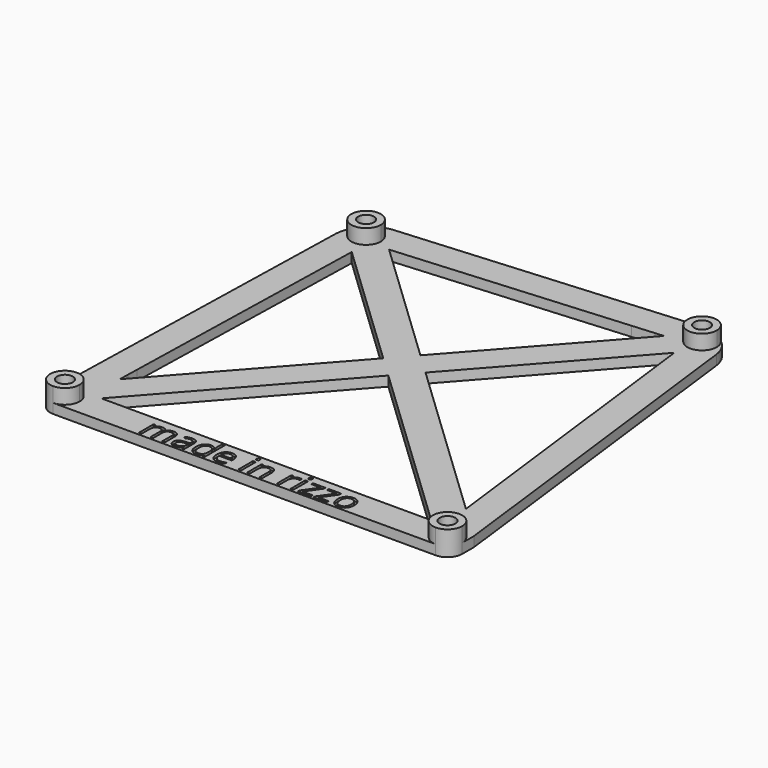
from build123d import *

# Parameters (mm, degrees)
F0_R         = 1.6
F1_DEPTH     = 2
F2_DEPTH     = 5
F3_TEXT_SIZE = 6.9444444444
F4_DEPTH     = 0.5
F5_T1_DEPTH  = 17
F6_R         = 6


# Not quite as in the source:
# - a fillet or chamfer that OpenCascade refuses, or shapes differently, is made with other operations: its cross-section is extruded or revolved along the edge and cut away or added
# - Text() gives the source's letters only with a copy of the font that has no kerning and outlines rounded to 1/6400 em; it was checked with that copy


with BuildPart() as f1:
    # F0 (on Top) → F1 (new body)
    with BuildSketch(Plane.XY):
        with BuildLine():
            ThreePointArc((-28.2406208698, -22.2661183476), (-29.1193005262, -24.3874386912), (-31.2406208698, -25.2661183476))
            Line((-31.2406208698, -25.2661183476), (46.7593791156, -25.2661183476))
            ThreePointArc((46.7593791156, -25.2661183476), (44.6380587918, -20.1447979989), (49.7593791302, -22.2661183476))
            Line((49.7593791302, -22.2661183476), (49.7593791302, -19.2661183476))
            Line((49.7593791302, -19.2661183476), (40.4943682456, 55.9885720374))
            Line((40.4943682456, 55.9885720374), (38.2495285372, 57.9787213655))
            Line((38.2495285372, 57.9787213655), (36.0046887452, 59.9688707678))
            Line((36.0046887452, 59.9688707678), (-28.3482573611, 54.975156742))
            Line((-28.3482573611, 54.975156742), (-30.4150766022, 52.8007010126))
            Line((-30.4150766022, 52.8007010126), (-32.4818959594, 50.626245161))
            Line((-32.4818959594, 50.626245161), (-34.2406208698, -19.2661183476))
            Line((-34.2406208698, -19.2661183476), (-34.2406208698, -22.2661183476))
            ThreePointArc((-34.2406208698, -22.2661183476), (-31.2406208698, -19.2661183476), (-28.2406208698, -22.2661183476))
        make_face()
        Polygon((0.1904056561, 19.5712364447), (-28.0633893681, -12.2983524785), (-28.0115448824, -10.2380338825), (-27.9546075256, -7.9753227447), (-26.6201953034, 45.0547011937), align=None, mode=Mode.SUBTRACT)
        Polygon((41.0503449115, -19.2661183476), (-26.2222311392, -19.2661183476), (4.5419359349, 15.4351087752), align=None, mode=Mode.SUBTRACT)
        with BuildLine():
            ThreePointArc((-25.2406208698, 50.7338816524), (-29.3534175275, 47.947901825), (-30.4150766022, 52.8007010126))
            ThreePointArc((-30.4150766022, 52.8007010126), (-27.1278242121, 53.5198614797), (-25.2406208698, 50.7338816524))
        make_face(mode=Mode.SUBTRACT)
        Polygon((30.2752796771, 53.5062376378), (4.1731011241, 24.0636194064), (-22.4946955335, 49.4113487276), (24.0214723183, 53.0209494356), (28.5091969851, 53.369191668), align=None, mode=Mode.SUBTRACT)
        Polygon((8.5246314029, 19.927491737), (35.1862162354, 50.0011065531), (41.8464502059, -4.0963847057), (42.3014974253, -7.7924880384), (42.9128945903, -12.7585377197), align=None, mode=Mode.SUBTRACT)
        with BuildLine():
            ThreePointArc((39.2593791302, 55.7338816524), (33.5234653687, 54.5031193319), (38.2495285372, 57.9787213655))
            ThreePointArc((38.2495285372, 57.9787213655), (38.9952928917, 56.9646439728), (39.2593791302, 55.7338816524))
        make_face(mode=Mode.SUBTRACT)
        with BuildLine():
            ThreePointArc((39.2593791302, 55.7338816524), (38.9952928917, 56.9646439728), (38.2495285372, 57.9787213655))
            ThreePointArc((38.2495285372, 57.9787213655), (33.5234653687, 54.5031193319), (39.2593791302, 55.7338816524))
        make_face()
        with Locations((36.2593791302, 55.7338816524)):
            Circle(F0_R, mode=Mode.SUBTRACT)
        with BuildLine():
            ThreePointArc((-25.2406208698, 50.7338816524), (-27.1278242121, 53.5198614797), (-30.4150766022, 52.8007010126))
            ThreePointArc((-30.4150766022, 52.8007010126), (-29.3534175275, 47.947901825), (-25.2406208698, 50.7338816524))
        make_face()
        with Locations((-28.2406208698, 50.7338816524)):
            Circle(F0_R, mode=Mode.SUBTRACT)
        with BuildLine():
            ThreePointArc((-34.2406208698, -22.2661183476), (-33.3619412134, -24.3874386912), (-31.2406208698, -25.2661183476))
            ThreePointArc((-31.2406208698, -25.2661183476), (-29.1193005262, -24.3874386912), (-28.2406208698, -22.2661183476))
            ThreePointArc((-28.2406208698, -22.2661183476), (-31.2406208698, -19.2661183476), (-34.2406208698, -22.2661183476))
        make_face()
        with Locations((-31.2406208698, -22.2661183476)):
            Circle(F0_R, mode=Mode.SUBTRACT)
        with BuildLine():
            ThreePointArc((49.7593791302, -22.2661183476), (44.6380587918, -20.1447979989), (46.7593791156, -25.2661183476))
            ThreePointArc((46.7593791156, -25.2661183476), (48.8806994686, -24.3874386964), (49.7593791302, -22.2661183476))
        make_face()
        with Locations((46.7593791302, -22.2661183476)):
            Circle(F0_R, mode=Mode.SUBTRACT)
        with BuildLine():
            Line((-34.2406208698, -22.2661183476), (-34.2406208698, -25.2661183476))
            Line((-34.2406208698, -25.2661183476), (-31.2406208698, -25.2661183476))
            ThreePointArc((-31.2406208698, -25.2661183476), (-33.3619412134, -24.3874386912), (-34.2406208698, -22.2661183476))
        make_face()
        with BuildLine():
            ThreePointArc((49.7593791302, -22.2661183476), (48.8806994686, -24.3874386964), (46.7593791156, -25.2661183476))
            Line((46.7593791156, -25.2661183476), (49.7593791302, -25.2661183476))
            Line((49.7593791302, -25.2661183476), (49.7593791302, -22.2661183476))
        make_face()
    extrude(amount=F1_DEPTH)

    # F0 (on Top) → F2 (join)
    with BuildSketch(Plane.XY):
        with BuildLine():
            ThreePointArc((-34.2406208698, -22.2661183476), (-33.3619412134, -24.3874386912), (-31.2406208698, -25.2661183476))
            ThreePointArc((-31.2406208698, -25.2661183476), (-29.1193005262, -24.3874386912), (-28.2406208698, -22.2661183476))
            ThreePointArc((-28.2406208698, -22.2661183476), (-31.2406208698, -19.2661183476), (-34.2406208698, -22.2661183476))
        make_face()
        with Locations((-31.2406208698, -22.2661183476)):
            Circle(F0_R, mode=Mode.SUBTRACT)
        with BuildLine():
            ThreePointArc((-25.2406208698, 50.7338816524), (-27.1278242121, 53.5198614797), (-30.4150766022, 52.8007010126))
            ThreePointArc((-30.4150766022, 52.8007010126), (-29.3534175275, 47.947901825), (-25.2406208698, 50.7338816524))
        make_face()
        with Locations((-28.2406208698, 50.7338816524)):
            Circle(F0_R, mode=Mode.SUBTRACT)
        with BuildLine():
            ThreePointArc((39.2593791302, 55.7338816524), (38.9952928917, 56.9646439728), (38.2495285372, 57.9787213655))
            ThreePointArc((38.2495285372, 57.9787213655), (33.5234653687, 54.5031193319), (39.2593791302, 55.7338816524))
        make_face()
        with Locations((36.2593791302, 55.7338816524)):
            Circle(F0_R, mode=Mode.SUBTRACT)
        with BuildLine():
            ThreePointArc((49.7593791302, -22.2661183476), (44.6380587918, -20.1447979989), (46.7593791156, -25.2661183476))
            ThreePointArc((46.7593791156, -25.2661183476), (48.8806994686, -24.3874386964), (49.7593791302, -22.2661183476))
        make_face()
        with Locations((46.7593791302, -22.2661183476)):
            Circle(F0_R, mode=Mode.SUBTRACT)
    extrude(amount=F2_DEPTH)

    # F3 (on face) → F4 (cut)
    with BuildSketch(Plane.XY.offset(2)):
        with Locations((-14.7463004105, -24.7661183476)):
            Text('made in rizzo', F3_TEXT_SIZE, font='Open Sans', text_align=(TextAlign.LEFT, TextAlign.BOTTOM))
    extrude(amount=-F4_DEPTH, mode=Mode.SUBTRACT)

    # F5: fillet of radius 3 on 2 edges, made by hand

    # F5_s2 → F5_t1 (cut)
    with BuildSketch(Plane.XY.offset(-7.5)):
        with BuildLine():
            ThreePointArc((-31.2406208698, -25.2661183476), (-33.3619412134, -24.3874386912), (-34.2406208698, -22.2661183476))
            Line((-34.2406208698, -22.2661183476), (-34.2406208698, -25.2661183476))
            Line((-34.2406208698, -25.2661183476), (-31.2406208698, -25.2661183476))
        make_face()
        with BuildLine():
            ThreePointArc((46.7593791302, -25.2661183476), (48.8806994738, -24.3874386912), (49.7593791302, -22.2661183476))
            Line((49.7593791302, -22.2661183476), (49.7593791302, -25.2661183476))
            Line((49.7593791302, -25.2661183476), (46.7593791302, -25.2661183476))
        make_face()
    extrude(amount=F5_T1_DEPTH, mode=Mode.SUBTRACT)

    # F6
    f6_edges = [f1.edges().sort_by_distance(p)[0] for p in [
        (-32.481896, 50.626245, 1),
        (-28.348257, 54.975157, 1),
        (36.004689, 59.968871, 1),
        (40.494368, 55.988572, 1),
    ]]
    fillet(f6_edges, radius=F6_R)


solid = f1.part
